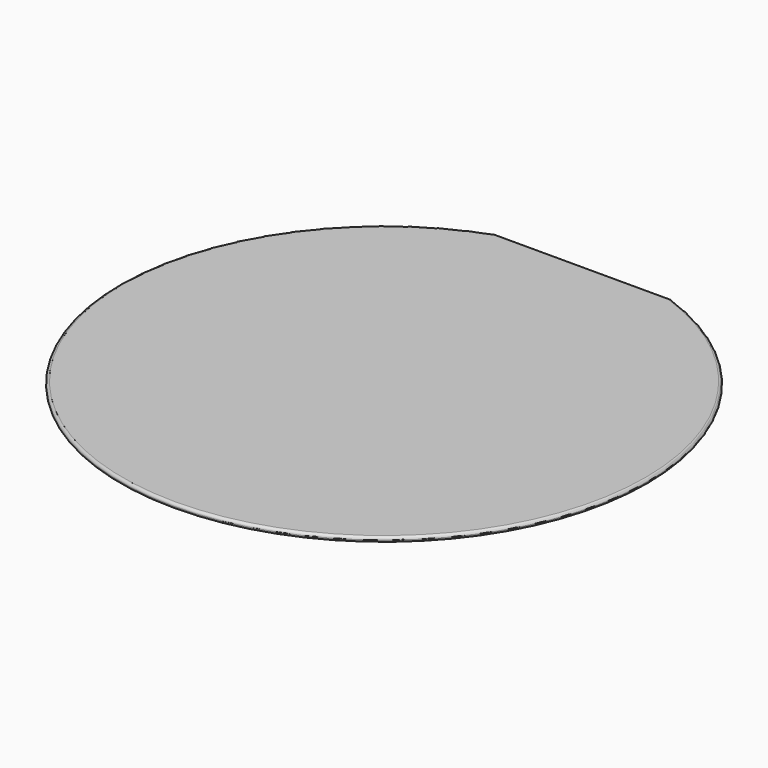
from build123d import *

# Parameters (mm, degrees)
F1_DEPTH = 1
F2_R     = 0.49999


# Not quite as in the source:
# - a fillet or chamfer is up to 0.001 mm smaller than in the source, because OpenCascade refuses the exact size


with BuildPart() as f1:
    # F0 (on Top) → F1 (new body)
    with BuildSketch(Plane.XY):
        with BuildLine():
            Line((16.6633232089, 47.1416340365), (-16.6633232089, 47.1416340365))
            ThreePointArc((-16.6633232089, 47.1416340365), (0, -50), (16.6633232089, 47.1416340365))
        make_face()
    extrude(amount=F1_DEPTH)

    # F2 (radius 0.5 in the source; OpenCascade refuses exactly that, so slightly less here)
    f2_edges = [f1.edges().sort_by_distance(p)[0] for p in [
        (0, 47.141634, 1),
        (0, -50, 1),
        (0, 47.141634, 0),
        (0, -50, 0),
    ]]
    fillet(f2_edges, radius=F2_R)


solid = f1.part
